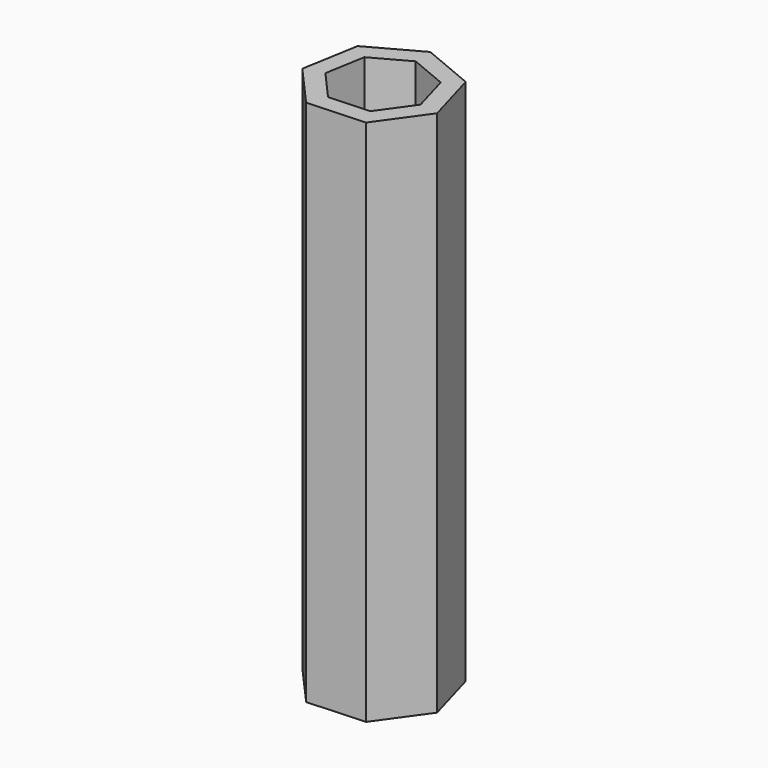
from build123d import *

# Parameters (mm, degrees)
F1_DEPTH = 304.8
F2_T     = -10.16


# Not quite as in the source:
# - a length typed as a fraction of an inch, garbled in the dataset ("3 / 203.2 mm" for 3/8 in), is restored


with BuildPart() as f1:
    # F0 (on Top) → F1 (new body)
    with BuildSketch(Plane.XY):
        Polygon((-9.5800449151, 1.4236958328), (-38.7624735933, -14.5894044641), (-44.4378743236, -47.3891506708), (-22.332554599, -72.2766649008), (10.9077289615, -70.5111413261), (30.2523648586, -43.4220552086), (21.1344477032, -11.4080409114), align=None)
    extrude(amount=-F1_DEPTH)

    # F2
    f2_openings = [f1.faces().sort_by_distance(p)[0] for p in [
        (-7.545487, -36.881823, 0),
    ]]
    offset(amount=F2_T, openings=f2_openings)


solid = f1.part
